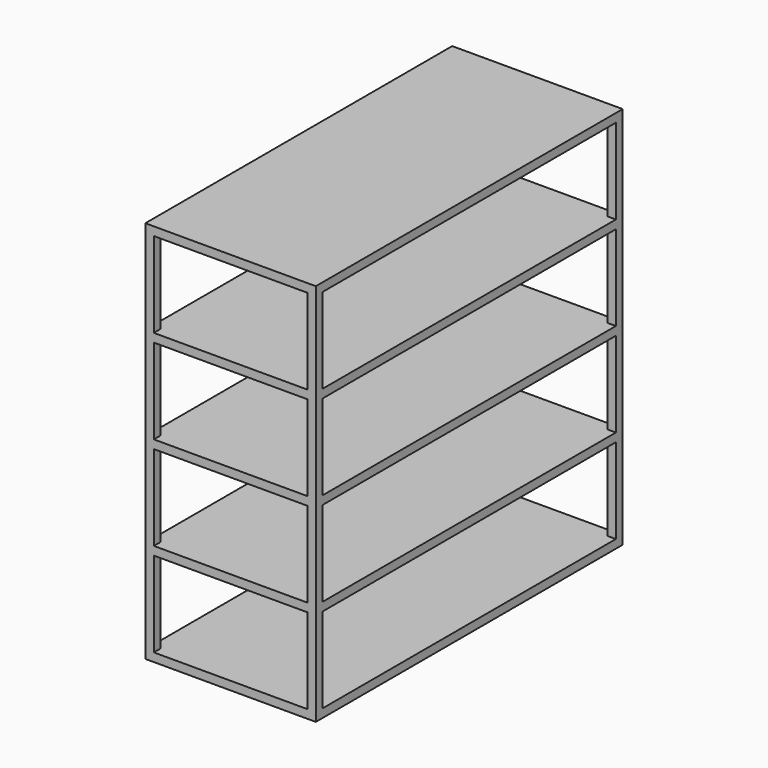
from build123d import *

# Parameters (mm, degrees)
F0_W     = 90
F0_H     = 40
F1_DEPTH = 90
F2_ANGLE = 90
F3_W     = 86
F3_H     = 20
F4_DEPTH = 40.001
F5_W     = 36
F5_H     = 20
F6_DEPTH = 90.001


# Not quite as in the source:
# - a feature names something its author has since deleted; it is built from what else it names


with BuildPart() as f1:
    # F0 (on Top) → F1 (new body)
    with BuildSketch(Plane.XY):
        with Locations((-1.7447127029, -1.7198646705)):
            Rectangle(F0_W, F0_H)
    extrude(amount=F1_DEPTH)


with BuildPart() as f1_1:
    # F2: moved
    add(f1.part.rotate(Axis((43.2552872971, 18.2801353295, 45), (0, 0, -1)), F2_ANGLE))

    # F3 (on face) → F4 (cut, through all)
    with BuildSketch(Plane.YZ.offset(43.2552872971)):
        with Locations((63.2801353295, 78)):
            Rectangle(F3_W, F3_H)
        with Locations((63.2801353295, 56)):
            Rectangle(F3_W, F3_H)
        with Locations((63.2801353295, 34)):
            Rectangle(F3_W, F3_H)
        with Locations((63.2801353295, 12)):
            Rectangle(F3_W, F3_H)
    extrude(amount=-F4_DEPTH, mode=Mode.SUBTRACT)

    # F5 (on face) → F6 (cut, through all)
    with BuildSketch(Plane.XZ.offset(-18.2801353295)):
        with Locations((23.2552872971, 78)):
            Rectangle(F5_W, F5_H)
        with Locations((23.2552872971, 56)):
            Rectangle(F5_W, F5_H)
        with Locations((23.2552872971, 34)):
            Rectangle(F5_W, F5_H)
        with Locations((23.2552872971, 12)):
            Rectangle(F5_W, F5_H)
    extrude(amount=-F6_DEPTH, mode=Mode.SUBTRACT)


solid = f1_1.part
